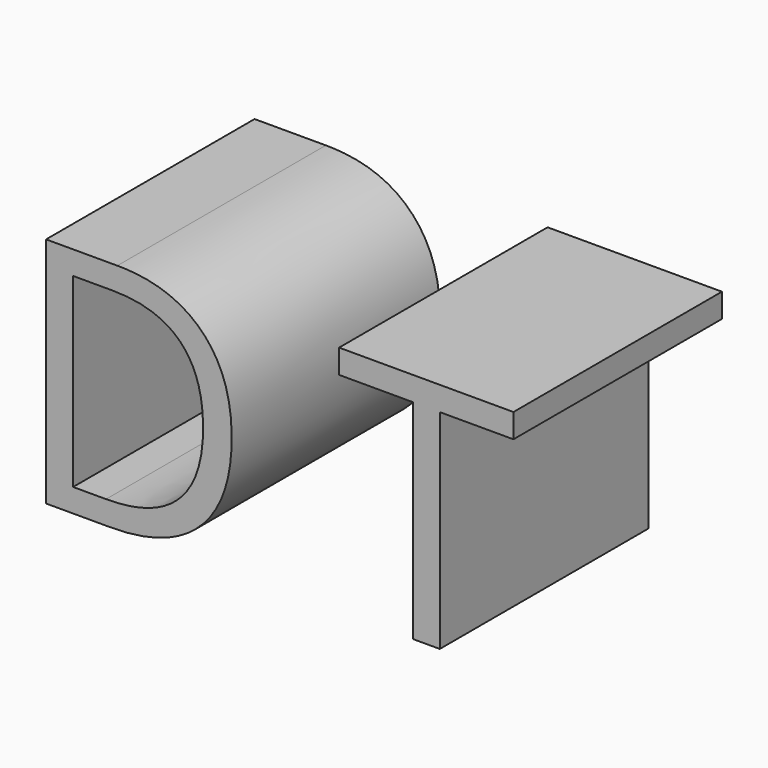
from build123d import *

# Parameters (mm, degrees)
F0_TEXT_SIZE = 31.75
F1_DEPTH     = 25.4


# Not quite as in the source:
# - Text() gives the source's letters only with a copy of the font that has no kerning and outlines rounded to 1/6400 em; it was checked with that copy


with BuildPart() as f1:
    # F0 (on Front) → F1 (new body)
    with BuildSketch(Plane.XZ):
        with Locations((-25.4805777277, -12.9371048097)):
            Text('D T', F0_TEXT_SIZE, font='Open Sans', text_align=(TextAlign.LEFT, TextAlign.BOTTOM))
    extrude(amount=F1_DEPTH)


solid = f1.part
